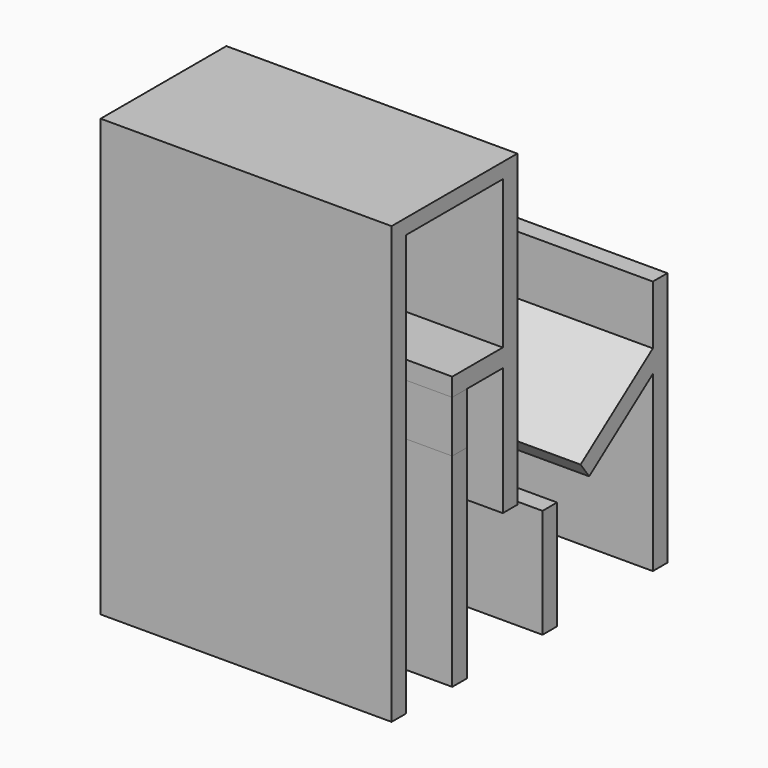
from build123d import *

# Parameters (mm, degrees)
F0_W     = 5
F0_H     = 35.0891035924
F1_DEPTH = 40
F0_H_2   = 30
F2_DEPTH = 2.5
F3_DEPTH = 40
F0_W_2   = 15.8472226467
F0_H_3   = 5
F4_DEPTH = 40


# Not quite as in the source:
# - a feature names something its author has since deleted; it is built from what else it names


with BuildPart() as f1:
    # F0 (on Right) → F1 (new body, symmetric)
    with BuildSketch(Plane.YZ):
        Polygon((13.9119866523, 115.8329709044), (13.9119866523, 120), (-24.2988105118, 120), (-24.2988105118, 115.8329709044), (-19.2988105118, 115.8329709044), align=None)
        Polygon((-24.2988105118, 0), (-19.2988105118, 0), (-19.2988105118, 16.3352508098), (-19.2988105118, 70.0891035924), (-19.2988105118, 75.0891035924), (-19.2988105118, 115.8329709044), (-24.2988105118, 115.8329709044), align=None)
        Polygon((13.9119866523, 70.0891035924), (18.9119866523, 70.0891035924), (18.9119866523, 120), (13.9119866523, 120), (13.9119866523, 115.8329709044), (13.9119866523, 75.0891035924), align=None)
        with Locations((16.4119866523, 52.5445517962)):
            Rectangle(F0_W, F0_H)
        Polygon((0, 70.0891035924), (1.5484121349, 70.0891035924), (13.9119866523, 70.0891035924), (13.9119866523, 75.0891035924), (-3.4515878651, 75.0891035924), (-3.4515878651, 70.0891035924), align=None)
    extrude(amount=F1_DEPTH, both=True)


with BuildPart() as f1b:
    # F0 (on Right) → F1, piece 2 (new body, symmetric)
    with BuildSketch(Plane.YZ):
        with Locations((30.0722406902, 15)):
            Rectangle(F0_W, F0_H_2)
    extrude(amount=F1_DEPTH, both=True)


with BuildPart() as f1c:
    # F0 (on Right) → F1, piece 3 (new body, symmetric)
    with BuildSketch(Plane.YZ):
        Polygon((65.4894374425, 53.9165928793), (40.6623113469, 35.8779891774), (43.6013059356, 31.8329538491), (65.4894374425, 47.7361771423), align=None)
        Polygon((65.4894374425, 47.7361771423), (65.4894374425, 0), (70.4894374425, 0), (70.4894374425, 53.9366312392), (70.4894374425, 70.0891035924), (65.4894374425, 70.0891035924), (65.4894374425, 53.9165928793), align=None)
    extrude(amount=F1_DEPTH, both=True)


with BuildPart() as f1d:
    # F0 (on Right) → F1, piece 4 (new body, symmetric)
    with BuildSketch(Plane.YZ):
        Polygon((-3.4515878651, 0), (1.5484121349, 0), (1.5484121349, 55.8824166656), (-3.4515878651, 55.8824166656), (-3.4515878651, 16.3352508098), align=None)
    extrude(amount=F1_DEPTH, both=True)


with BuildPart() as f2:
    # F0 (on Right) → F2 (new body, symmetric)
    with BuildSketch(Plane.YZ):
        Polygon((-3.4515878651, 55.8824166656), (1.5484121349, 55.8824166656), (1.5484121349, 70.0891035924), (0, 70.0891035924), (-3.4515878651, 70.0891035924), align=None)
        Polygon((-19.2988105118, 16.3352508098), (-3.4515878651, 16.3352508098), (-3.4515878651, 55.8824166656), (-3.4515878651, 70.0891035924), (-19.2988105118, 70.0891035924), align=None)
    extrude(amount=F2_DEPTH, both=True)


with BuildPart() as f3:
    # F0 (on Right) → F3 (new body, through all)
    with BuildSketch(Plane.YZ):
        Polygon((-3.4515878651, 55.8824166656), (1.5484121349, 55.8824166656), (1.5484121349, 70.0891035924), (0, 70.0891035924), (-3.4515878651, 70.0891035924), align=None)
    extrude(amount=F3_DEPTH)


with BuildPart() as f4:
    # F0 (on Right) → F4 (new body, through all)
    with BuildSketch(Plane.YZ):
        with Locations((-11.3751991885, 72.5891035924)):
            Rectangle(F0_W_2, F0_H_3)
    extrude(amount=-F4_DEPTH)


solid = Compound([f1.part, f1b.part, f1c.part, f1d.part, f2.part, f3.part, f4.part])
